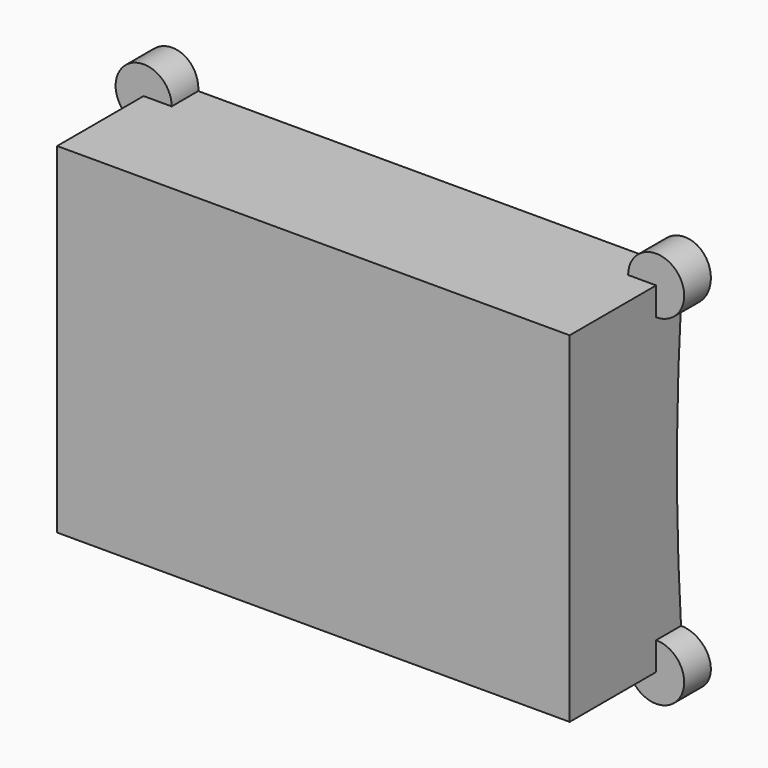
from build123d import *

# Parameters (mm, degrees)
F1_DEPTH  = 46.99
F2_T      = -3.175
F5_DEPTH  = 12.7
F6_R      = 635
F7_DEPTH  = 279.4
F8_DEPTH  = 3.175
F9_W      = 137.16
F9_H      = 3.175
F10_DEPTH = 19.05


# Not quite as in the source:
# - a feature names something its author has since deleted; it is built from what else it names


with BuildPart() as f1:
    # F0 (on Front) → F1 (new body)
    with BuildSketch(Plane.XZ):
        Polygon((-72.39, 53.975), (-81.28, 53.975), (-81.28, 45.085), (-81.28, -45.085), (-81.28, -53.975), (-72.39, -53.975), (72.39, -53.975), (81.28, -53.975), (81.28, -45.085), (81.28, 45.085), (81.28, 53.975), (72.39, 53.975), align=None)
    extrude(amount=F1_DEPTH)

    # F2
    f2_openings = [f1.faces().sort_by_distance(p)[0] for p in [
        (0, 0, 0),
    ]]
    offset(amount=F2_T, openings=f2_openings)

    # F0 (on Front) → F5 (join)
    with BuildSketch(Plane.XZ):
        with BuildLine():
            Line((-81.28, 45.085), (-81.28, 53.975))
            Line((-81.28, 53.975), (-72.39, 53.975))
            ThreePointArc((-72.39, 53.975), (-87.5661792847, 60.2611792847), (-81.28, 45.085))
        make_face()
        with BuildLine():
            Line((-81.28, -53.975), (-81.28, -45.085))
            ThreePointArc((-81.28, -45.085), (-87.5661792847, -60.2611792847), (-72.39, -53.975))
            Line((-72.39, -53.975), (-81.28, -53.975))
        make_face()
        with BuildLine():
            ThreePointArc((81.28, 45.085), (87.5661792847, 60.2611792847), (72.39, 53.975))
            Line((72.39, 53.975), (81.28, 53.975))
            Line((81.28, 53.975), (81.28, 45.085))
        make_face()
        with BuildLine():
            ThreePointArc((72.39, -53.975), (87.5661792847, -60.2611792847), (81.28, -45.085))
            Line((81.28, -45.085), (81.28, -53.975))
            Line((81.28, -53.975), (72.39, -53.975))
        make_face()
    extrude(amount=F5_DEPTH)

    # F6 (on offset) → F7 (cut)
    with BuildSketch(Plane(origin=(-106.68, 0, 0), x_dir=(0, -1, 0), z_dir=(-1, 0, 0))):
        with Locations((-630.555, 0)):
            Circle(F6_R)
    extrude(amount=-F7_DEPTH, mode=Mode.SUBTRACT)

    # F4 (on face) → F8 (cut)
    with BuildSketch(Plane(origin=(-81.28, 0, 0), x_dir=(0, -1, 0), z_dir=(-1, 0, 0))):
        Polygon((24.13, 0), (13.97, 0), (3.81, 0), (3.81, -6.35), (24.13, -6.35), align=None)
        Polygon((3.81, 0), (13.97, 0), (24.13, 0), (24.13, 6.35), (3.81, 6.35), align=None)
    extrude(amount=-F8_DEPTH, mode=Mode.SUBTRACT)

    # F9 (on face) → F10 (join)
    with BuildSketch(Plane(origin=(0, -43.815, 0), x_dir=(-1, 0, 0), z_dir=(0, 1, 0))):
        with Locations((-9.525, -1.5875)):
            Rectangle(F9_W, F9_H)
        with Locations((-9.525, 1.5875)):
            Rectangle(F9_W, F9_H)
    extrude(amount=F10_DEPTH)


solid = f1.part
